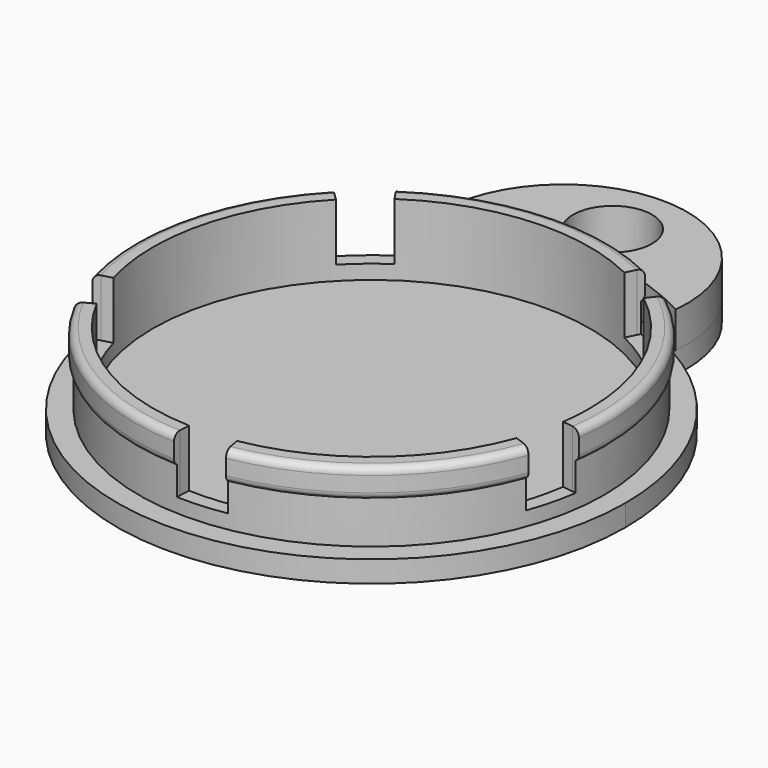
from build123d import *

# Parameters (mm, degrees)
F0_R      = 2.75
F1_DEPTH  = 1.5
F2_R      = 16.25
F2_R_2    = 15.25
F3_DEPTH  = 3
F4_R      = 2.75
F5_DEPTH  = 2.5
F6_R      = 16.5
F6_R_2    = 16.25
F6_R_3    = 15.25
F7_DEPTH  = 2
F10_DEPTH = 4
F11_R     = 0.5


# Not quite as in the source:
# - a fillet or chamfer that OpenCascade refuses, or shapes differently, is made with other operations: its cross-section is extruded or revolved along the edge and cut away or added


with BuildPart() as f1:
    # F0 (on Top) → F1 (new body)
    with BuildSketch(Plane.XY):
        with BuildLine():
            ThreePointArc((-8.5809247648, 15.5380252986), (-9.0208393574, -15.2868229952), (17.75, 0))
            ThreePointArc((17.75, 0), (15.2868229952, 9.0208393574), (8.5809247648, 15.5380252986))
            ThreePointArc((8.5809247648, 15.5380252986), (0, 17.75), (-8.5809247648, 15.5380252986))
        make_face()
        with BuildLine():
            ThreePointArc((-8.5809247648, 15.5380252986), (0, 17.75), (8.5809247648, 15.5380252986))
            ThreePointArc((8.5809247648, 15.5380252986), (6.5344178783, 22.4200078248), (0, 25.3951140277))
            ThreePointArc((0, 25.3951140277), (-6.5344178783, 22.4200078248), (-8.5809247648, 15.5380252986))
        make_face()
        with Locations((0, 21.05)):
            Circle(F0_R, mode=Mode.SUBTRACT)
    extrude(amount=F1_DEPTH)

    # F2 (on face) → F3 (join)
    with BuildSketch(Plane.XY.offset(1.5)):
        Circle(F2_R)
        Circle(F2_R_2, mode=Mode.SUBTRACT)
    extrude(amount=F3_DEPTH)

    # F4 (on face) → F5 (join)
    with BuildSketch(Plane.XY.offset(1.5)):
        with BuildLine():
            ThreePointArc((-8.612627735, 15.7937710626), (9.10413e-05, 17.9970129536), (8.6124927052, 15.7925318064))
            ThreePointArc((8.6124927052, 15.7925318064), (0.0006232955, 25.3951140053), (-8.612627735, 15.7937710626))
        make_face()
        with Locations((0, 21.05)):
            Circle(F4_R, mode=Mode.SUBTRACT)
    extrude(amount=F5_DEPTH)

    # F6 (on face) → F7 (join)
    with BuildSketch(Plane.XY.offset(4.5)):
        Circle(F6_R)
        Circle(F6_R_2, mode=Mode.SUBTRACT)
        Circle(F6_R_2)
        Circle(F6_R_3, mode=Mode.SUBTRACT)
    extrude(amount=F7_DEPTH)

    # F8: fillet of radius 0.5 on 2 edges, made by hand

    # F8_s1 → F8_t2 (revolve, cut)
    with BuildSketch(Plane.XZ):
        with BuildLine():
            ThreePointArc((16.5, 6), (16.3535533906, 6.3535533906), (16, 6.5))
            Line((16, 6.5), (16.5, 6.5))
            Line((16.5, 6.5), (16.5, 6))
        make_face()
    revolve(axis=Axis((0, 0, 6.5), (0, 0, 1)), mode=Mode.SUBTRACT)

    # F8_s3 → F8_t4 (revolve, cut)
    with BuildSketch(Plane.XZ):
        with BuildLine():
            ThreePointArc((16.25, 4.5), (16.4330127019, 4.6830127019), (16.5, 4.9330127019))
            Line((16.5, 4.9330127019), (16.5, 4.5))
            Line((16.5, 4.5), (16.25, 4.5))
        make_face()
    revolve(axis=Axis((0, 0, 4.5), (0, 0, 1)), mode=Mode.SUBTRACT)

    # F9 (on face) → F10 (cut)
    with BuildSketch(Plane.XY.offset(6.5)):
        with BuildLine():
            Line((7.0301885691, 14.3727676069), (6.7006484799, 13.6990441254))
            ThreePointArc((6.7006484799, 13.6990441254), (8.0958816571, 12.9235908398), (9.4024146607, 12.0065439885))
            Line((9.4024146607, 12.0065439885), (9.8648284964, 12.5970297585))
            ThreePointArc((9.8648284964, 12.5970297585), (8.4940397714, 13.5591772745), (7.0301885691, 14.3727676069))
        make_face()
        with BuildLine():
            Line((7.6425660227, 15.6247338583), (7.0301885691, 14.3727676069))
            ThreePointArc((7.0301885691, 14.3727676069), (8.4940397714, 13.5591772745), (9.8648284964, 12.5970297585))
            Line((9.8648284964, 12.5970297585), (10.7241224536, 13.6943171116))
            Line((10.7241224536, 13.6943171116), (7.6425660227, 15.6247338583))
        make_face()
        with BuildLine():
            Line((15.8417620313, -2.2446772027), (15.0991794361, -2.1394579588))
            ThreePointArc((15.0991794361, -2.1394579588), (14.7928302986, -3.7060318073), (14.3244078168, -5.2320015958))
            Line((14.3244078168, -5.2320015958), (15.0288868898, -5.4893131497))
            ThreePointArc((15.0288868898, -5.4893131497), (15.5203465428, -3.8882956667), (15.8417620313, -2.2446772027))
        make_face()
        with BuildLine():
            Line((17.2216877329, -2.4402039223), (15.8417620313, -2.2446772027))
            ThreePointArc((15.8417620313, -2.2446772027), (15.5203465428, -3.8882956667), (15.0288868898, -5.4893131497))
            Line((15.0288868898, -5.4893131497), (16.3380056131, -5.9674698272))
            Line((16.3380056131, -5.9674698272), (17.2216877329, -2.4402039223))
        make_face()
        with BuildLine():
            Line((2.7605588079, -15.760054412), (2.6311576138, -15.0213018614))
            ThreePointArc((2.6311576138, -15.0213018614), (1.0465902573, -15.2140444601), (-0.5494437612, -15.2400988039))
            Line((-0.5494437612, -15.2400988039), (-0.5764655855, -15.9896118599))
            ThreePointArc((-0.5764655855, -15.9896118599), (1.0980619093, -15.9622761548), (2.7605588079, -15.760054412))
        make_face()
        with BuildLine():
            Line((3.0010223399, -17.1328628218), (2.7605588079, -15.760054412))
            ThreePointArc((2.7605588079, -15.760054412), (1.0980619093, -15.9622761548), (-0.5764655855, -15.9896118599))
            Line((-0.5764655855, -15.9896118599), (-0.6266796763, -17.3824162917))
            Line((-0.6266796763, -17.3824162917), (3.0010223399, -17.1328628218))
        make_face()
        with BuildLine():
            Line((-14.13564286, -7.4955720885), (-13.473034601, -7.1442171468))
            ThreePointArc((-13.473034601, -7.1442171468), (-14.1460019473, -5.6967647754), (-14.6639827361, -4.186897457))
            Line((-14.6639827361, -4.186897457), (-15.3851622149, -4.3928104466))
            ThreePointArc((-15.3851622149, -4.3928104466), (-14.8417069611, -5.9769335348), (-14.13564286, -7.4955720885))
        make_face()
        with BuildLine():
            Line((-15.3851622149, -4.3928104466), (-16.7253149532, -4.7754542476))
            Line((-16.7253149532, -4.7754542476), (-15.3669539259, -8.1484876261))
            Line((-15.3669539259, -8.1484876261), (-14.13564286, -7.4955720885))
            ThreePointArc((-14.13564286, -7.4955720885), (-14.8417069611, -5.9769335348), (-15.3851622149, -4.3928104466))
        make_face()
        with BuildLine():
            ThreePointArc((-8.9320875858, 13.2747056977), (-10.2707412623, 12.2683280818), (-11.4968665483, 11.1275360962))
            Line((-11.4968665483, 11.1275360962), (-10.9579509288, 10.6059328416))
            ThreePointArc((-10.9579509288, 10.6059328416), (-9.7893002656, 11.693250203), (-8.5133959802, 12.6524538681))
            Line((-8.5133959802, 12.6524538681), (-8.9320875858, 13.2747056977))
        make_face()
        with BuildLine():
            Line((-9.7101334373, 14.4310232549), (-12.4983221696, 12.0968205119))
            Line((-12.4983221696, 12.0968205119), (-11.4968665483, 11.1275360962))
            ThreePointArc((-11.4968665483, 11.1275360962), (-10.2707412623, 12.2683280818), (-8.9320875858, 13.2747056977))
            Line((-8.9320875858, 13.2747056977), (-9.7101334373, 14.4310232549))
        make_face()
    extrude(amount=-F10_DEPTH, mode=Mode.SUBTRACT)

    # F11
    f11_edges = [f1.edges().sort_by_distance(p)[0] for p in [
        (-2.75, 21.05, 0),
    ]]
    fillet(f11_edges, radius=F11_R)


solid = f1.part
